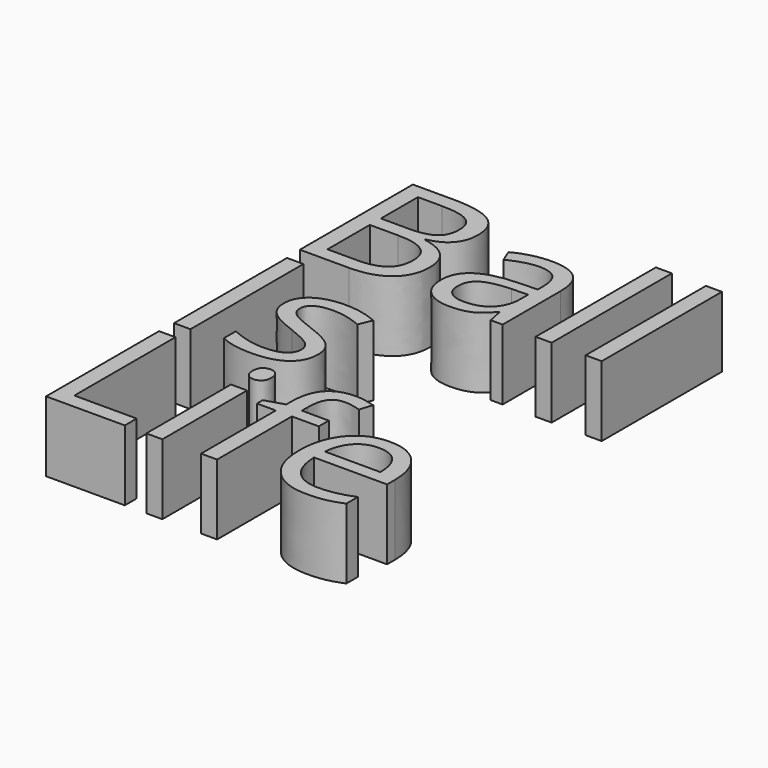
from build123d import *

# Parameters (mm, degrees)
F0_TEXT_SIZE = 29.9861111111
F3_DEPTH     = 10.668
F1_TEXT_SIZE = 29.9861111111
F4_DEPTH     = 10.668
F2_TEXT_SIZE = 29.9861111111
F5_DEPTH     = 10.668


# Not quite as in the source:
# - Text() gives the source's letters only with a copy of the font that has no kerning and outlines rounded to 1/6400 em; it was checked with that copy


with BuildPart() as f3:
    # F0 (on Top) → F3 (new body)
    with BuildSketch(Plane.XY):
        with Locations((-68.6035904691, 25.6487759431)):
            Text('Ball', F0_TEXT_SIZE, font='Open Sans', text_align=(TextAlign.LEFT, TextAlign.BOTTOM))
    extrude(amount=F3_DEPTH)


with BuildPart() as f4:
    # F1 (on Top) → F4 (new body)
    with BuildSketch(Plane.XY):
        with Locations((-68.477099579, 1.6404452467)):
            Text('Is', F1_TEXT_SIZE, font='Open Sans', text_align=(TextAlign.LEFT, TextAlign.BOTTOM))
    extrude(amount=F4_DEPTH)


with BuildPart() as f5:
    # F2 (on Top) → F5 (new body)
    with BuildSketch(Plane.XY):
        with Locations((-68.5809069546, -22.4799208917)):
            Text('Life', F2_TEXT_SIZE, font='Open Sans', text_align=(TextAlign.LEFT, TextAlign.BOTTOM))
    extrude(amount=F5_DEPTH)


solid = Compound([f3.part, f4.part, f5.part])
